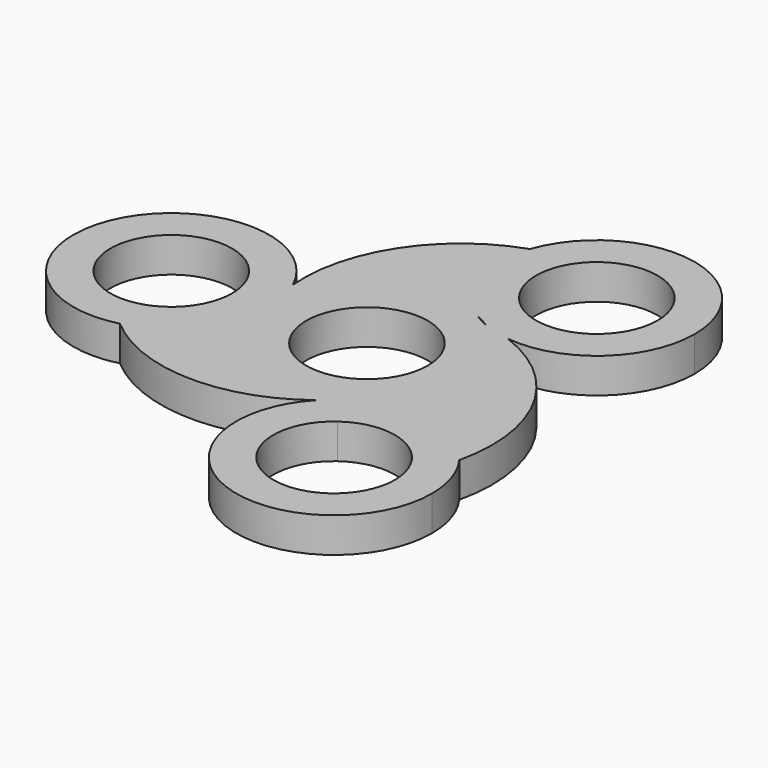
from build123d import *

# Parameters (mm, degrees)
F0_R     = 11.049
F1_DEPTH = 6.35


with BuildPart() as f1:
    # F0 (on Top) → F1 (new body)
    with BuildSketch(Plane.XY):
        with BuildLine():
            ThreePointArc((10.5094277958, -14.3415594481), (15.8585312405, -8.0396136036), (17.78, 0))
            ThreePointArc((17.78, 0), (15.6108797336, 8.5105131421), (9.6327745846, 14.9444991151))
            ThreePointArc((9.6327745846, 14.9444991151), (8.3729133787, 15.5596772314), (7.1654409141, 16.2722111745))
            ThreePointArc((7.1654409141, 16.2722111745), (-9.7140841192, 14.8917752376), (-17.78, 0))
            ThreePointArc((-17.78, 0), (-9.4273906442, -15.0749031719), (7.7827340428, -15.986164356))
            ThreePointArc((7.7827340428, -15.986164356), (9.1091896886, -15.102697614), (10.5094277958, -14.3415594481))
        make_face()
        Circle(F0_R, mode=Mode.SUBTRACT)
        with BuildLine():
            ThreePointArc((9.6327745846, 14.9444991151), (15.6108797336, 8.5105131421), (17.78, 0))
            ThreePointArc((17.78, 0), (15.8585312405, -8.0396136036), (10.5094277958, -14.3415594481))
            ThreePointArc((10.5094277958, -14.3415594481), (22.5963149024, -13.0765595999), (32.6723306155, -19.8711877644))
            ThreePointArc((32.6723306155, -19.8711877644), (30.024905988, 0.2187336146), (14.766870478, 13.5531308843))
            ThreePointArc((14.766870478, 13.5531308843), (12.1474957403, 14.0557311296), (9.6327745846, 14.9444991151))
        make_face()
        with BuildLine():
            ThreePointArc((14.766870478, 13.5531308843), (12.2321244934, 14.3680080122), (9.6327745846, 14.9444991151))
            ThreePointArc((9.6327745846, 14.9444991151), (12.1474957403, 14.0557311296), (14.766870478, 13.5531308843))
        make_face()
        with BuildLine():
            ThreePointArc((7.1654409141, 16.2722111745), (8.42530212, 15.6570330582), (9.6327745846, 14.9444991151))
            ThreePointArc((9.6327745846, 14.9444991151), (12.2321244934, 14.3680080122), (14.766870478, 13.5531308843))
            ThreePointArc((14.766870478, 13.5531308843), (28.6306092872, 17.9455815797), (34.5782154987, 31.2167102896))
            ThreePointArc((34.5782154987, 31.2167102896), (19.7525452394, 48.7495462206), (0, 37.0432320702))
            ThreePointArc((0, 37.0432320702), (-0.0097628586, 25.4184119581), (7.1654409141, 16.2722111745))
        make_face()
        with BuildLine():
            ThreePointArc((27.8472154987, 31.2167102896), (22.8348249156, 21.9625356777), (12.3454057878, 21.1046933455))
            ThreePointArc((12.3454057878, 21.1046933455), (10.7616060818, 40.4708849015), (27.8472154987, 31.2167102896))
        make_face(mode=Mode.SUBTRACT)
        with BuildLine():
            ThreePointArc((32.6723306155, -19.8711877644), (22.5963149024, -13.0765595999), (10.5094277958, -14.3415594481))
            ThreePointArc((10.5094277958, -14.3415594481), (9.1829721501, -15.2250261902), (7.7827340428, -15.986164356))
            ThreePointArc((7.7827340428, -15.986164356), (6.6242894769, -17.0632176818), (5.4082696447, -18.0748171313))
            ThreePointArc((5.4082696447, -18.0748171313), (11.6947079059, -46.8383870739), (36.0721618387, -30.3277238042))
            ThreePointArc((36.0721618387, -30.3277238042), (35.2008548818, -24.8300425135), (32.6723306155, -19.8711877644))
        make_face()
        with BuildLine():
            ThreePointArc((29.3411618387, -30.3277238042), (13.2961162421, -40.1826682179), (11.761303137, -21.4154690043))
            ThreePointArc((11.761303137, -21.4154690043), (23.2882074352, -20.4727793905), (29.3411618387, -30.3277238042))
        make_face(mode=Mode.SUBTRACT)
        with BuildLine():
            ThreePointArc((7.7827340428, -15.986164356), (9.1829721501, -15.2250261902), (10.5094277958, -14.3415594481))
            ThreePointArc((10.5094277958, -14.3415594481), (9.1091896886, -15.102697614), (7.7827340428, -15.986164356))
        make_face()
        with BuildLine():
            ThreePointArc((-17.78, 0), (-9.7140841192, 14.8917752376), (7.1654409141, 16.2722111745))
            ThreePointArc((7.1654409141, 16.2722111745), (-0.0097628586, 25.4184119581), (0, 37.0432320702))
            ThreePointArc((0, 37.0432320702), (-14.8117955692, 25.6039367366), (-19.4235623734, 7.4661757763))
            ThreePointArc((-19.4235623734, 7.4661757763), (-18.1957513695, 3.8224690318), (-17.78, 0))
        make_face()
        with BuildLine():
            ThreePointArc((5.4082696447, -18.0748171313), (6.5489734879, -16.9775954393), (7.7827340428, -15.986164356))
            ThreePointArc((7.7827340428, -15.986164356), (-9.4273906442, -15.0749031719), (-17.78, 0))
            ThreePointArc((-17.78, 0), (-21.5036758006, -10.8879819067), (-31.115, -17.2154109739))
            ThreePointArc((-31.115, -17.2154109739), (-13.0077535924, -24.206353637), (5.4082696447, -18.0748171313))
        make_face()
        with BuildLine():
            ThreePointArc((5.4082696447, -18.0748171313), (6.6242894769, -17.0632176818), (7.7827340428, -15.986164356))
            ThreePointArc((7.7827340428, -15.986164356), (6.5489734879, -16.9775954393), (5.4082696447, -18.0748171313))
        make_face()
        with BuildLine():
            ThreePointArc((-19.4235623734, 7.4661757763), (-18.851475509, 3.67812157), (-17.78, 0))
            ThreePointArc((-17.78, 0), (-18.1957513695, 3.8224690318), (-19.4235623734, 7.4661757763))
        make_face()
        with BuildLine():
            ThreePointArc((-31.115, -17.2154109739), (-21.5036758006, -10.8879819067), (-17.78, 0))
            ThreePointArc((-17.78, 0), (-18.851475509, 3.67812157), (-19.4235623734, 7.4661757763))
            ThreePointArc((-19.4235623734, 7.4661757763), (-51.6284185538, 7.6114601214), (-31.115, -17.2154109739))
        make_face()
        with Locations((-35.56, 0)):
            Circle(F0_R, mode=Mode.SUBTRACT)
    extrude(amount=F1_DEPTH)


solid = f1.part
